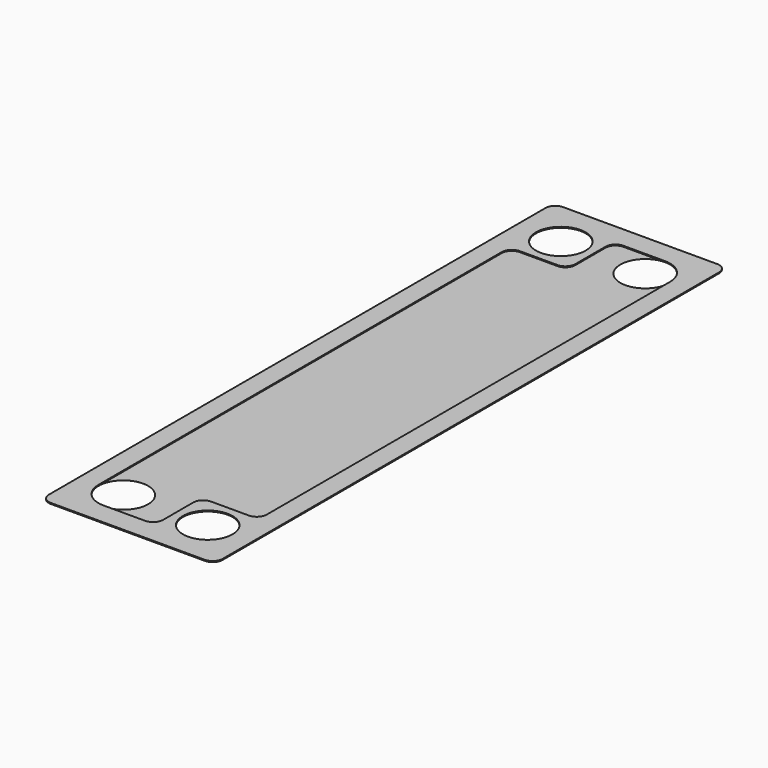
from build123d import *

# Parameters (mm, degrees)
F0_W     = 88.9
F0_H     = 327.66
F0_R     = 12.7
F0_R_2   = 12.7063161154
F1_DEPTH = 0.5
F2_DEPTH = 0.005
F3_R     = 5.08
F4_R     = 5.08


# Not quite as in the source:
# - a feature names something its author has since deleted; it is built from what else it names


with BuildPart() as f1:
    # F0 (on Top) → F1 (new body)
    with BuildSketch(Plane.XY):
        with Locations((-16.0019993782, 26.0465461761)):
            Rectangle(F0_W, F0_H)
        with Locations((5.5880006218, -113.6534538239)):
            Circle(F0_R, mode=Mode.SUBTRACT)
        with Locations((-37.5932163954, 166.1064843748)):
            Circle(F0_R_2, mode=Mode.SUBTRACT)
        with BuildLine():
            ThreePointArc((5.589217639, 178.8128004902), (14.573939928, 175.0912066639), (18.2955337543, 166.1064843748))
            Line((18.2955337543, 166.1064843748), (18.2955337543, -96.8894538239))
            Line((18.2955337543, -96.8894538239), (-11.1759993782, -96.8894538239))
            Line((-11.1759993782, -96.8894538239), (-11.1759993782, -126.3534538239))
            Line((-11.1759993782, -126.3534538239), (-37.5919993782, -126.3534538239))
            ThreePointArc((-37.5919993782, -126.3534538239), (-46.5722554993, -122.633709945), (-50.2919993782, -113.6534538239))
            Line((-50.2919993782, -113.6534538239), (-50.2919993782, 149.3424895761))
            Line((-50.2919993782, 149.3424895761), (-20.826782361, 149.3424895761))
            Line((-20.826782361, 149.3424895761), (-20.826782361, 178.8128004902))
            Line((-20.826782361, 178.8128004902), (5.589217639, 178.8128004902))
        make_face(mode=Mode.SUBTRACT)
    extrude(amount=F1_DEPTH)

    # F0 (on Top) → F2 (join)
    with BuildSketch(Plane.XY):
        with BuildLine():
            Line((18.2955337543, -96.8894538239), (18.2955337543, 166.1064843748))
            ThreePointArc((18.2955337543, 166.1064843748), (-3.3955046501, 157.1217620858), (5.589217639, 178.8128004902))
            Line((5.589217639, 178.8128004902), (-20.826782361, 178.8128004902))
            Line((-20.826782361, 178.8128004902), (-20.826782361, 149.3424895761))
            Line((-20.826782361, 149.3424895761), (-50.2919993782, 149.3424895761))
            Line((-50.2919993782, 149.3424895761), (-50.2919993782, -113.6534538239))
            ThreePointArc((-50.2919993782, -113.6534538239), (-37.5919993782, -100.9534538239), (-24.8919993782, -113.6534538239))
            ThreePointArc((-24.8919993782, -113.6534538239), (-28.6117432571, -122.633709945), (-37.5919993782, -126.3534538239))
            Line((-37.5919993782, -126.3534538239), (-11.1759993782, -126.3534538239))
            Line((-11.1759993782, -126.3534538239), (-11.1759993782, -96.8894538239))
            Line((-11.1759993782, -96.8894538239), (18.2955337543, -96.8894538239))
        make_face()
    extrude(amount=F2_DEPTH)

    # F3
    f3_edges = [f1.edges().sort_by_distance(p)[0] for p in [
        (28.448001, 189.876546, 0.25),
        (-60.451999, 189.876546, 0.25),
        (-60.451999, -137.783454, 0.25),
        (28.448001, -137.783454, 0.25),
        (18.295534, -96.889454, 0.2525),
        (-11.175999, -96.889454, 0.2525),
        (-11.175999, -126.353454, 0.2525),
    ]]
    fillet(f3_edges, radius=F3_R)

    # F4
    f4_edges = [f1.edges().sort_by_distance(p)[0] for p in [
        (-20.826782, 149.34249, 0.2525),
        (-50.291999, 149.34249, 0.2525),
        (-20.826782, 178.8128, 0.2525),
    ]]
    fillet(f4_edges, radius=F4_R)


solid = f1.part
